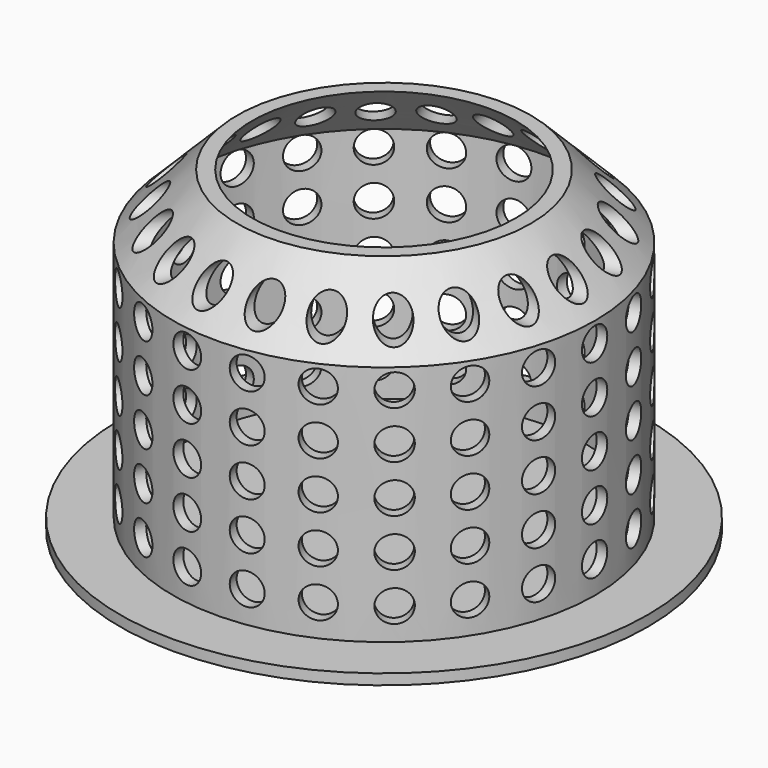
from build123d import *

# Parameters (mm, degrees)
F0_R             = 20
F1_DEPTH         = 30
F2_SIZE          = 6.1
F3_R             = 25
F4_DEPTH         = 1
F5_T             = -1
F6_R             = 1.5
F7_DEPTH         = 40
F7_COPIES1_COUNT = 11
F7_COPIES1_ANGLE = 163.6363636364
F7_COPIES2_COUNT = 11
F7_COPIES2_ANGLE = 163.6363636364


# Not quite as in the source:
# - a pattern or mirror of a feature is missing from the dataset's text; its kind, count and spacing are read off the source's solid


with BuildPart() as f1:
    # F0 (on Top) → F1 (new body)
    with BuildSketch(Plane.XY):
        Circle(F0_R)
    extrude(amount=F1_DEPTH)

    # F2
    f2_edges = [f1.edges().sort_by_distance(p)[0] for p in [
        (-20, 0, 30),
    ]]
    chamfer(f2_edges, length=F2_SIZE)

    # F3 (on Top) → F4 (join)
    with BuildSketch(Plane.XY):
        Circle(F3_R)
    extrude(amount=F4_DEPTH)

    # F5
    f5_openings = [f1.faces().sort_by_distance(p)[0] for p in [
        (0, 0, 30),
    ]]
    offset(amount=F5_T, openings=f5_openings, kind=Kind.INTERSECTION)

    # F6 (on Right) → F7 (cut)
    with BuildSketch(Plane.YZ):
        with Locations((0, 4)):
            Circle(F6_R)
        with Locations((0, 8.5)):
            Circle(F6_R)
        with Locations((0, 13)):
            Circle(F6_R)
        with Locations((0, 17.5)):
            Circle(F6_R)
        with Locations((0, 22)):
            Circle(F6_R)
        with Locations((0, 26.5)):
            Circle(F6_R)
    f7 = extrude(amount=-F7_DEPTH, mode=Mode.SUBTRACT)

    # F7_copies: F7 across plane
    add(f7.mirror(Plane(origin=(0, 0, 0), x_dir=(0, 0, 1), z_dir=(1, 0, 0))), mode=Mode.SUBTRACT)

    # F7_copies1: F7 ×11 about axis
    f7_copies1_axis = Axis((0, 0, 0), (0, 0, 1))
    for i in range(1, F7_COPIES1_COUNT):
        add(f7.rotate(f7_copies1_axis, i * F7_COPIES1_ANGLE / (F7_COPIES1_COUNT - 1)), mode=Mode.SUBTRACT)

    # F7_copies2: F7 ×11 about axis
    f7_copies2_axis = Axis((0, 0, 0), (0, 0, -1))
    for i in range(1, F7_COPIES2_COUNT):
        add(f7.rotate(f7_copies2_axis, i * F7_COPIES2_ANGLE / (F7_COPIES2_COUNT - 1)), mode=Mode.SUBTRACT)


solid = f1.part
